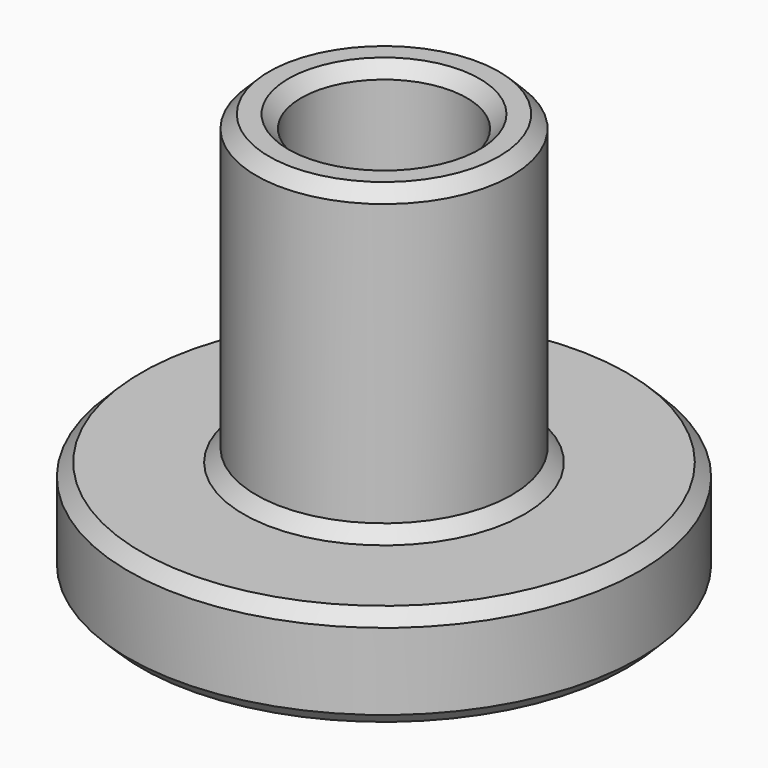
from build123d import *

# Parameters (mm, degrees)
F0_R     = 15.875
F1_DEPTH = 25.4
F2_D     = 10.3
F3_SIZE  = 0.79375
F4_SIZE  = 0.79375
F5_R     = 15.875
F5_R_2   = 7.9375
F6_DEPTH = 19.05
F7_SIZE  = 0.79375


with BuildPart() as f1:
    # F0 (on Top) → F1 (new body)
    with BuildSketch(Plane.XY):
        Circle(F0_R)
    extrude(amount=F1_DEPTH)

    # F2 (through all)
    with Locations(Plane(origin=(0, 0, 0), x_dir=(1, 0, 0), z_dir=(0, 0, -1))):
        with Locations((0, 0)):
            Hole(F2_D / 2)

    # F3
    f3_edges = [f1.edges().sort_by_distance(p)[0] for p in [
        (-15.875, 0, 0),
    ]]
    chamfer(f3_edges, length=F3_SIZE)

    # F4
    f4_edges = [f1.edges().sort_by_distance(p)[0] for p in [
        (-15.875, 0, 25.4),
        (-5.15, 0, 25.4),
        (-5.15, 0, 0),
    ]]
    chamfer(f4_edges, length=F4_SIZE)

    # F5 (on face) → F6 (cut)
    with BuildSketch(Plane.XY.offset(25.4)):
        Circle(F5_R)
        Circle(F5_R_2, mode=Mode.SUBTRACT)
    extrude(amount=-F6_DEPTH, mode=Mode.SUBTRACT)

    # F7
    f7_edges = [f1.edges().sort_by_distance(p)[0] for p in [
        (-15.875, 0, 6.35),
        (-7.9375, 0, 6.35),
        (-7.9375, 0, 25.4),
    ]]
    chamfer(f7_edges, length=F7_SIZE)


solid = f1.part
